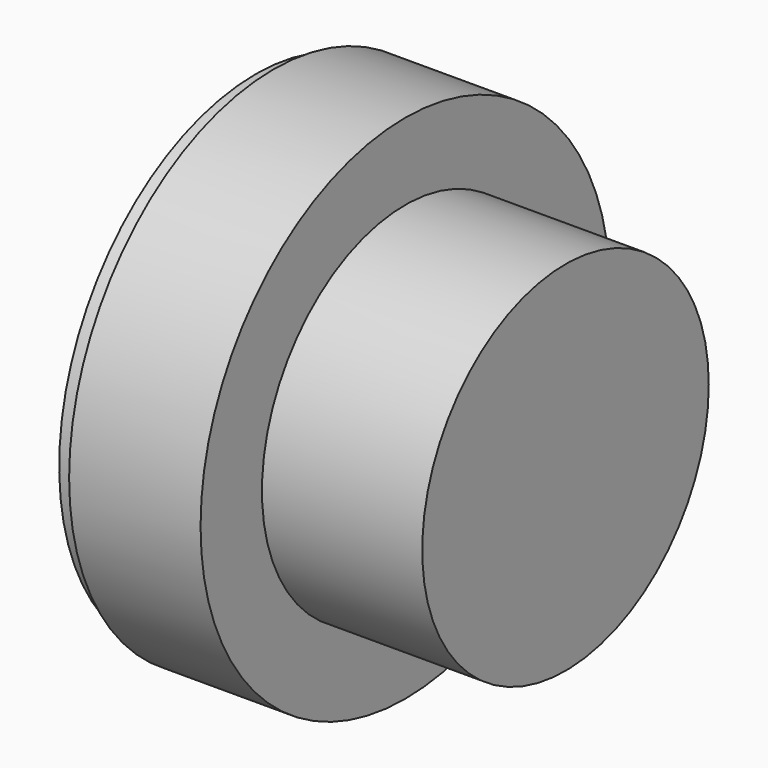
from build123d import *

# Parameters (mm, degrees)
F2_R     = 88.9
F4_DEPTH = 127


# Not quite as in the source:
# - the program builds the solid bodies; features that only make, move or delete a surface that nothing else refers to are left out


with BuildPart() as f1:
    # F0 (on Front) → F1 (revolve)
    with BuildSketch(Plane.XZ):
        Polygon((-17.8278337446, 25.4), (0, 25.4), (55.6368945653, 25.4), (55.6368945653, 50.8), (47.4307299643, 50.8), (47.4307299643, 127), (-17.8278337446, 127), (-17.8278337446, 121.92), (-26.8155404944, 121.92), (-26.8155404944, 30.48), (-17.8278337446, 30.48), align=None)
    revolve(axis=Axis((17.3414491085, 0, 0), (1, 0, 0)))

    # F2 (on Right) → F4 (join)
    with BuildSketch(Plane.YZ):
        Circle(F2_R)
    extrude(amount=F4_DEPTH)


solid = f1.part
